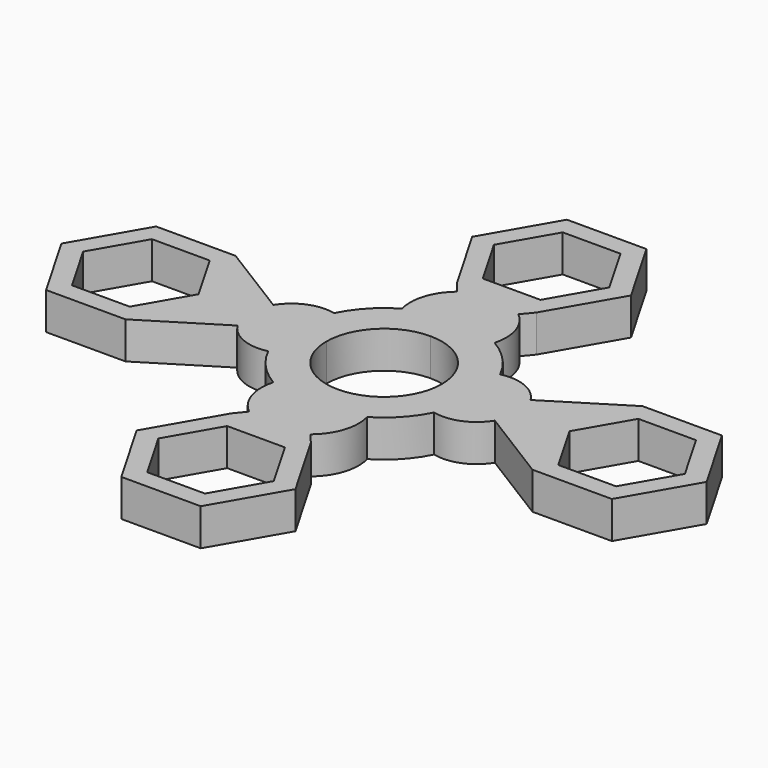
from build123d import *

# Parameters (mm, degrees)
F1_DEPTH = 7


# Not quite as in the source:
# - a feature names something its author has since deleted; it is built from what else it names


with BuildPart() as f1:
    # F0 (on Top) → F1 (new body)
    with BuildSketch(Plane.XY):
        Polygon((-53.4446571767, -12.9903810568), (-38.4446571767, -12.9903810568), (-30.9446571767, 0), (-38.4446571767, 12.9903810568), (-53.4446571767, 12.9903810568), (-60.9446571767, 0), align=None)
        Polygon((-56.8446571767, 0), (-51.3946571767, 9.4396769013), (-40.4946571767, 9.4396769013), (-35.0446571767, 0), (-40.4946571767, -9.4396769013), (-51.3946571767, -9.4396769013), align=None, mode=Mode.SUBTRACT)
        with BuildLine():
            ThreePointArc((0, 10.9), (7.7074639149, 7.7074639149), (10.9, 0))
            Line((10.9, 0), (17.5, 0))
            ThreePointArc((17.5, 0), (17.0367250374, 4), (15.6714285714, 7.78821716))
            ThreePointArc((15.6714285714, 7.78821716), (12.7504247795, 11.9865202599), (8.7403572641, 15.1610077137))
            ThreePointArc((8.7403572641, 15.1610077137), (4.5239565101, 16.9051417473), (0, 17.5))
            Line((0, 17.5), (0, 10.9))
        make_face()
        with BuildLine():
            Line((17.5, 0), (10.9, 0))
            ThreePointArc((10.9, 0), (7.7074639149, -7.7074639149), (0, -10.9))
            Line((0, -10.9), (0, -17.5))
            ThreePointArc((0, -17.5), (4.5925968465, -16.8866235289), (8.8632518819, -15.0894919092))
            ThreePointArc((8.8632518819, -15.0894919092), (12.7990151761, -11.9346223452), (15.6714285714, -7.78821716))
            ThreePointArc((15.6714285714, -7.78821716), (17.0367250374, -4), (17.5, 0))
        make_face()
        with BuildLine():
            ThreePointArc((-10.9, 0), (-7.7074639149, 7.7074639149), (0, 10.9))
            Line((0, 10.9), (0, 17.5))
            ThreePointArc((0, 17.5), (-4.5239565101, 16.9051417473), (-8.7403572641, 15.1610077137))
            ThreePointArc((-8.7403572641, 15.1610077137), (-12.7504247795, 11.9865202599), (-15.6714285714, 7.78821716))
            ThreePointArc((-15.6714285714, 7.78821716), (-17.0367250374, 4), (-17.5, 0))
            Line((-17.5, 0), (-10.9, 0))
        make_face()
        Polygon((-7.5, 26.5479130202), (0, 26.5479130202), (7.5, 26.5479130202), (15, 39.5382940769), (7.5, 52.5286751337), (-7.5, 52.5286751337), (-15, 39.5382940769), align=None)
        Polygon((-10.9, 39.5382940769), (-5.45, 48.9779709782), (5.45, 48.9779709782), (10.9, 39.5382940769), (5.45, 30.0986171757), (-5.45, 30.0986171757), align=None, mode=Mode.SUBTRACT)
        Polygon((30.9, 0), (38.4, -12.9903810568), (53.4, -12.9903810568), (60.9, 0), (53.4, 12.9903810568), (38.4, 12.9903810568), align=None)
        Polygon((40.45, -9.4396769013), (35, 0), (40.45, 9.4396769013), (51.35, 9.4396769013), (56.8, 0), (51.35, -9.4396769013), align=None, mode=Mode.SUBTRACT)
        Polygon((7.5, -26.6851936929), (0, -26.6851936929), (-7.5, -26.6851936929), (-15, -39.6755747497), (-7.5, -52.6659558065), (7.5, -52.6659558065), (15, -39.6755747497), align=None)
        Polygon((-10.9, -39.6755747497), (-5.45, -30.2358978485), (5.45, -30.2358978485), (10.9, -39.6755747497), (5.45, -49.115251651), (-5.45, -49.115251651), align=None, mode=Mode.SUBTRACT)
        with BuildLine():
            Line((0, 26.5479130202), (0, 17.5))
            Line((0, 17.5), (5.7741715282, 24.4658935667))
            ThreePointArc((5.7741715282, 24.4658935667), (3.0690333104, 26.0115077724), (0, 26.5479130202))
        make_face()
        with BuildLine():
            Line((7.5, 26.5479130202), (0, 26.5479130202))
            ThreePointArc((0, 26.5479130202), (3.0690333104, 26.0115077724), (5.7741715282, 24.4658935667))
            Line((5.7741715282, 24.4658935667), (7.5, 26.5479130202))
        make_face()
        with BuildLine():
            ThreePointArc((-5.7741715282, 24.4658935667), (-3.0690333104, 26.0115077724), (0, 26.5479130202))
            Line((0, 26.5479130202), (-7.5, 26.5479130202))
            Line((-7.5, 26.5479130202), (-5.7741715282, 24.4658935667))
        make_face()
        with BuildLine():
            Line((-5.7741715282, 24.4658935667), (0, 17.5))
            Line((0, 17.5), (0, 26.5479130202))
            ThreePointArc((0, 26.5479130202), (-3.0690333104, 26.0115077724), (-5.7741715282, 24.4658935667))
        make_face()
        with BuildLine():
            Line((5.8093756333, -24.6146987236), (0, -17.5))
            Line((0, -17.5), (0, -26.6851936929))
            ThreePointArc((0, -26.6851936929), (3.0836583252, -26.1521000058), (5.8093756333, -24.6146987236))
        make_face()
        with BuildLine():
            ThreePointArc((5.8093756333, -24.6146987236), (3.0836583252, -26.1521000058), (0, -26.6851936929))
            Line((0, -26.6851936929), (7.5, -26.6851936929))
            Line((7.5, -26.6851936929), (5.8093756333, -24.6146987236))
        make_face()
        with BuildLine():
            Line((-7.5, -26.6851936929), (0, -26.6851936929))
            ThreePointArc((0, -26.6851936929), (-3.0836583252, -26.1521000058), (-5.8093756333, -24.6146987236))
            Line((-5.8093756333, -24.6146987236), (-7.5, -26.6851936929))
        make_face()
        with BuildLine():
            Line((0, -26.6851936929), (0, -17.5))
            Line((0, -17.5), (-5.8093756333, -24.6146987236))
            ThreePointArc((-5.8093756333, -24.6146987236), (-3.0836583252, -26.1521000058), (0, -26.6851936929))
        make_face()
        with BuildLine():
            Line((-38.4446571767, -12.9903810568), (-24.2985391386, -4.2166177892))
            ThreePointArc((-24.2985391386, -4.2166177892), (-25.1937738825, -2.1922234023), (-25.5, 0))
            Line((-25.5, 0), (-30.9446571767, 0))
            Line((-30.9446571767, 0), (-38.4446571767, -12.9903810568))
        make_face()
        with BuildLine():
            ThreePointArc((-25.5, 0), (-25.1937738825, 2.1922234023), (-24.2985391386, 4.2166177892))
            Line((-24.2985391386, 4.2166177892), (-38.4446571767, 12.9903810568))
            Line((-38.4446571767, 12.9903810568), (-30.9446571767, 0))
            Line((-30.9446571767, 0), (-25.5, 0))
        make_face()
        with BuildLine():
            ThreePointArc((25.5, 0), (25.1927245669, -2.1959027158), (24.2945028156, -4.2231186922))
            Line((24.2945028156, -4.2231186922), (38.4, -12.9903810568))
            Line((38.4, -12.9903810568), (30.9, 0))
            Line((30.9, 0), (25.5, 0))
        make_face()
        with BuildLine():
            Line((38.4, 12.9903810568), (24.2945028156, 4.2231186922))
            ThreePointArc((24.2945028156, 4.2231186922), (25.1927245669, 2.1959027158), (25.5, 0))
            Line((25.5, 0), (30.9, 0))
            Line((30.9, 0), (38.4, 12.9903810568))
        make_face()
        with BuildLine():
            Line((-24.2985391386, -4.2166177892), (-17.5, 0))
            Line((-17.5, 0), (-22.5, 0))
            Line((-22.5, 0), (-25.5, 0))
            ThreePointArc((-25.5, 0), (-25.1937738825, -2.1922234023), (-24.2985391386, -4.2166177892))
        make_face()
        with BuildLine():
            Line((-22.5, 0), (-17.5, 0))
            Line((-17.5, 0), (-24.2985391386, 4.2166177892))
            ThreePointArc((-24.2985391386, 4.2166177892), (-25.1937738825, 2.1922234023), (-25.5, 0))
            Line((-25.5, 0), (-22.5, 0))
        make_face()
        with BuildLine():
            Line((24.2945028156, 4.2231186922), (17.5, 0))
            Line((17.5, 0), (22.5, 0))
            Line((22.5, 0), (25.5, 0))
            ThreePointArc((25.5, 0), (25.1927245669, 2.1959027158), (24.2945028156, 4.2231186922))
        make_face()
        with BuildLine():
            Line((22.5, 0), (17.5, 0))
            Line((17.5, 0), (24.2945028156, -4.2231186922))
            ThreePointArc((24.2945028156, -4.2231186922), (25.1927245669, -2.1959027158), (25.5, 0))
            Line((25.5, 0), (22.5, 0))
        make_face()
        with BuildLine():
            Line((-5.8093756333, -24.6146987236), (0, -17.5))
            ThreePointArc((0, -17.5), (-4.5925968465, -16.8866235289), (-8.8632518819, -15.0894919092))
            ThreePointArc((-8.8632518819, -15.0894919092), (-8.7466502596, -20.3042632567), (-5.8093756333, -24.6146987236))
        make_face()
        with BuildLine():
            ThreePointArc((8.8632518819, -15.0894919092), (4.5925968465, -16.8866235289), (0, -17.5))
            Line((0, -17.5), (5.8093756333, -24.6146987236))
            ThreePointArc((5.8093756333, -24.6146987236), (8.7466502596, -20.3042632567), (8.8632518819, -15.0894919092))
        make_face()
        with BuildLine():
            Line((24.2945028156, -4.2231186922), (17.5, 0))
            ThreePointArc((17.5, 0), (17.0367250374, -4), (15.6714285714, -7.78821716))
            ThreePointArc((15.6714285714, -7.78821716), (20.5565667679, -7.3930642898), (24.2945028156, -4.2231186922))
        make_face()
        with BuildLine():
            ThreePointArc((15.6714285714, 7.78821716), (17.0367250374, 4), (17.5, 0))
            Line((17.5, 0), (24.2945028156, 4.2231186922))
            ThreePointArc((24.2945028156, 4.2231186922), (20.5565667679, 7.3930642898), (15.6714285714, 7.78821716))
        make_face()
        with BuildLine():
            ThreePointArc((-15.6714285714, -7.78821716), (-17.0367250374, -4), (-17.5, 0))
            Line((-17.5, 0), (-24.2985391386, -4.2166177892))
            ThreePointArc((-24.2985391386, -4.2166177892), (-20.5601021676, -7.3916016346), (-15.6714285714, -7.78821716))
        make_face()
        with BuildLine():
            Line((0, -17.5), (0, -10.9))
            ThreePointArc((0, -10.9), (-7.7074639149, -7.7074639149), (-10.9, 0))
            Line((-10.9, 0), (-17.5, 0))
            ThreePointArc((-17.5, 0), (-17.0367250374, -4), (-15.6714285714, -7.78821716))
            ThreePointArc((-15.6714285714, -7.78821716), (-12.7990151761, -11.9346223452), (-8.8632518819, -15.0894919092))
            ThreePointArc((-8.8632518819, -15.0894919092), (-4.5925968465, -16.8866235289), (0, -17.5))
        make_face()
        with BuildLine():
            Line((-24.2985391386, 4.2166177892), (-17.5, 0))
            ThreePointArc((-17.5, 0), (-17.0367250374, 4), (-15.6714285714, 7.78821716))
            ThreePointArc((-15.6714285714, 7.78821716), (-20.5601021676, 7.3916016346), (-24.2985391386, 4.2166177892))
        make_face()
        with BuildLine():
            ThreePointArc((-8.7403572641, 15.1610077137), (-4.5239565101, 16.9051417473), (0, 17.5))
            Line((0, 17.5), (-5.7741715282, 24.4658935667))
            ThreePointArc((-5.7741715282, 24.4658935667), (-8.6205053042, 20.2480208005), (-8.7403572641, 15.1610077137))
        make_face()
        with BuildLine():
            Line((5.7741715282, 24.4658935667), (0, 17.5))
            ThreePointArc((0, 17.5), (4.5239565101, 16.9051417473), (8.7403572641, 15.1610077137))
            ThreePointArc((8.7403572641, 15.1610077137), (8.6205053042, 20.2480208005), (5.7741715282, 24.4658935667))
        make_face()
    extrude(amount=F1_DEPTH)


solid = f1.part
